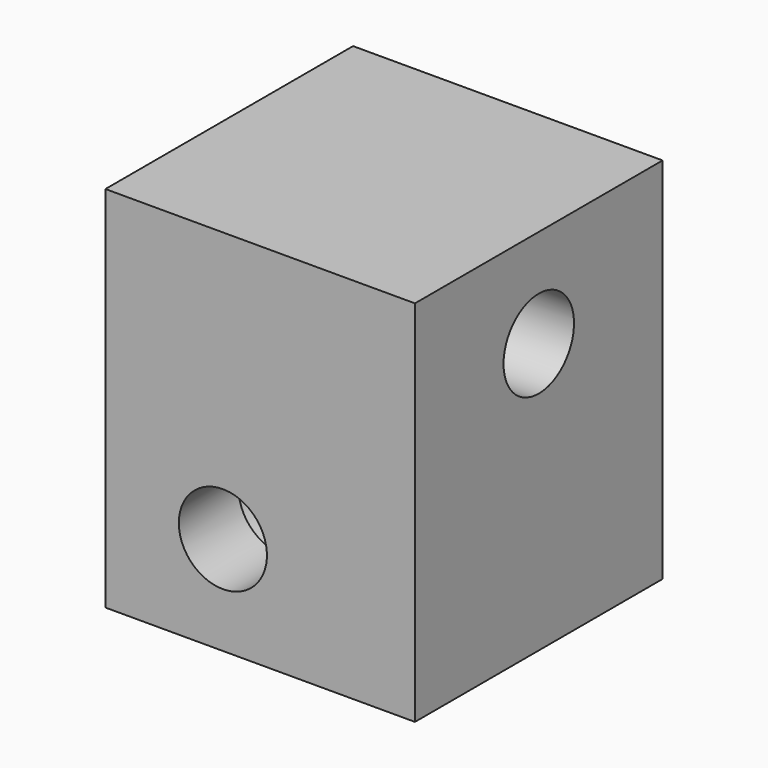
from build123d import *

# Parameters (mm, degrees)
F0_W      = 12.00023
F0_H      = 10.0584
F1_DEPTH  = 24.00046
F2_W      = 24.00046
F2_H      = 37.6428
F3_DEPTH  = 7.62
F4_W      = 31.62046
F4_H      = 37.6428
F4_R      = 7.5057
F5_DEPTH  = 7.62
F6_R      = 4.5
F7_DEPTH  = 25.4
F9_DEPTH  = 24.00046
F10_R     = 4.5
F11_DEPTH = 25.4


with BuildPart() as f1:
    # F0 (on Front) → F1 (new body)
    with BuildSketch(Plane.XZ):
        with BuildLine():
            Line((0, 10.0584), (0, 0))
            Line((0, 0), (12.00023, 0))
            Line((12.00023, 0), (12.00023, 2.5527))
            ThreePointArc((12.00023, 2.5527), (6.6928986324, 4.7510686324), (4.49453, 10.0584))
            Line((4.49453, 10.0584), (0, 10.0584))
        make_face()
        with BuildLine():
            Line((0, 27.5844), (0, 10.0584))
            Line((0, 10.0584), (4.49453, 10.0584))
            ThreePointArc((4.49453, 10.0584), (6.6928986324, 15.3657313676), (12.00023, 17.5641))
            Line((12.00023, 17.5641), (12.00023, 27.5844))
            Line((12.00023, 27.5844), (0, 27.5844))
        make_face()
        with Locations((6.000115, 32.6136)):
            Rectangle(F0_W, F0_H)
        with Locations((18.000345, 32.6136)):
            Rectangle(F0_W, F0_H)
        with BuildLine():
            Line((19.50593, 10.0584), (24.00046, 10.0584))
            Line((24.00046, 10.0584), (24.00046, 27.5844))
            Line((24.00046, 27.5844), (12.00023, 27.5844))
            Line((12.00023, 27.5844), (12.00023, 17.5641))
            ThreePointArc((12.00023, 17.5641), (17.3075613676, 15.3657313676), (19.50593, 10.0584))
        make_face()
        with BuildLine():
            Line((12.00023, 2.5527), (12.00023, 0))
            Line((12.00023, 0), (24.00046, 0))
            Line((24.00046, 0), (24.00046, 10.0584))
            Line((24.00046, 10.0584), (19.50593, 10.0584))
            ThreePointArc((19.50593, 10.0584), (17.3075613676, 4.7510686324), (12.00023, 2.5527))
        make_face()
    extrude(amount=F1_DEPTH)

    # F2 (on face) → F3 (join)
    with BuildSketch(Plane.YZ.offset(24.00046)):
        with Locations((-12.00023, 18.8214)):
            Rectangle(F2_W, F2_H)
    extrude(amount=F3_DEPTH)

    # F4 (on face) → F5 (join)
    with BuildSketch(Plane.XZ.offset(24.00046)):
        with Locations((15.81023, 18.8214)):
            Rectangle(F4_W, F4_H)
        with Locations((12.00023, 10.0584)):
            Circle(F4_R, mode=Mode.SUBTRACT)
        with Locations((12.00023, 10.0584)):
            Circle(F4_R)
    extrude(amount=F5_DEPTH)

    # F6 (on face) → F7 (cut)
    with BuildSketch(Plane(origin=(0, -24.00046, 0), x_dir=(-1, 0, 0), z_dir=(0, 1, 0))):
        with Locations((-12.00023, 10.0584)):
            Circle(F6_R)
    extrude(amount=-F7_DEPTH, mode=Mode.SUBTRACT)

    # F8 (on face) → F9 (cut)
    with BuildSketch(Plane(origin=(0, 0, 0), x_dir=(0, -1, 0), z_dir=(-1, 0, 0))):
        with BuildLine():
            ThreePointArc((8.30453, 27.5971), (15.81023, 20.0914), (23.31593, 27.5971))
            Line((23.31593, 27.5971), (15.81023, 27.5971))
            Line((15.81023, 27.5971), (8.30453, 27.5971))
        make_face()
        with BuildLine():
            Line((15.81023, 27.5971), (23.31593, 27.5971))
            ThreePointArc((23.31593, 27.5971), (15.81023, 35.1028), (8.30453, 27.5971))
            Line((8.30453, 27.5971), (15.81023, 27.5971))
        make_face()
    extrude(amount=-F9_DEPTH, mode=Mode.SUBTRACT)

    # F10 (on face) → F11 (cut)
    with BuildSketch(Plane(origin=(24.00046, 0, 0), x_dir=(0, -1, 0), z_dir=(-1, 0, 0))):
        with Locations((15.81023, 27.5971)):
            Circle(F10_R)
    extrude(amount=-F11_DEPTH, mode=Mode.SUBTRACT)


solid = f1.part
